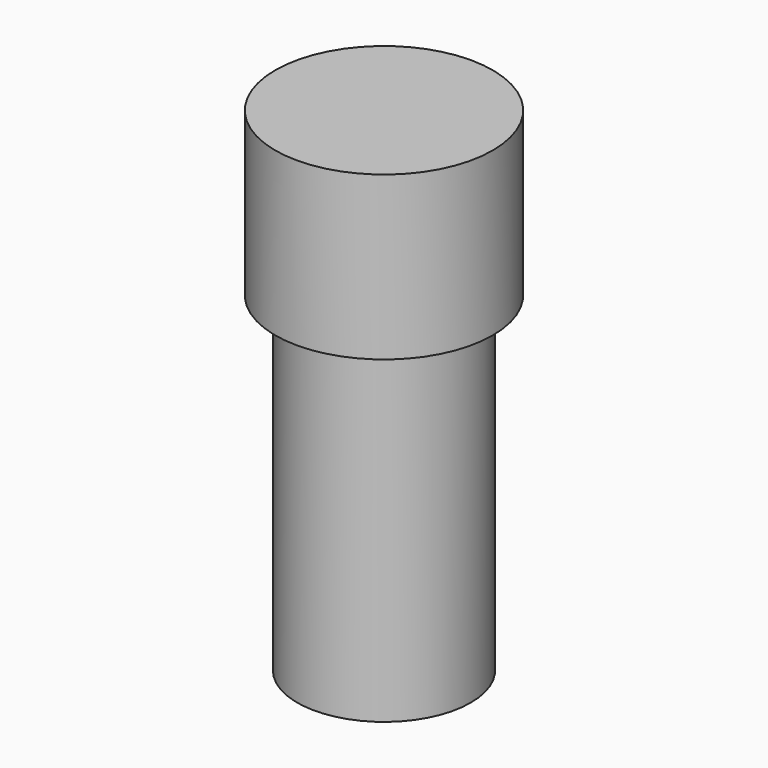
from build123d import *

# Parameters (mm, degrees)
F0_R     = 16.9607668537
F2_DEPTH = 25.4
F4_R     = 13.5349469598
F5_DEPTH = 51.562


# Not quite as in the source:
# - the program builds the solid bodies; features that only make, move or delete a surface that nothing else refers to are left out


with BuildPart() as f2:
    # F0 (on Top) → F2 (new body)
    with BuildSketch(Plane.XY):
        Circle(F0_R)
    extrude(amount=F2_DEPTH)

    # F4 (on Top) → F5 (join)
    with BuildSketch(Plane.XY):
        Circle(F4_R)
    extrude(amount=-F5_DEPTH)


solid = f2.part
